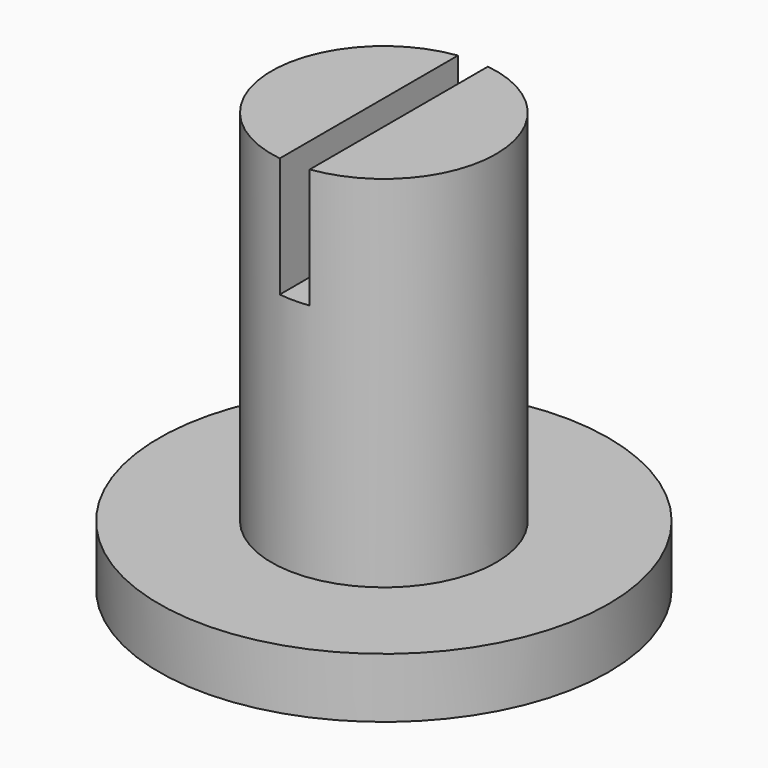
from build123d import *

# Parameters (mm, degrees)
F0_R     = 1.875
F1_DEPTH = 7
F0_R_2   = 3.75
F2_DEPTH = 1
F4_DEPTH = 2


with BuildPart() as f1:
    # F0 (on Top) → F1 (new body)
    with BuildSketch(Plane.XY):
        Circle(F0_R)
    extrude(amount=F1_DEPTH)

    # F0 (on Top) → F2 (join)
    with BuildSketch(Plane.XY):
        Circle(F0_R_2)
        Circle(F0_R, mode=Mode.SUBTRACT)
    extrude(amount=F2_DEPTH)

    # F3 (on face) → F4 (cut)
    with BuildSketch(Plane.XY.offset(7)):
        with BuildLine():
            Line((-0.25, 1.8582585934), (-0.25, -1.8582585934))
            ThreePointArc((-0.25, -1.8582585934), (0, -1.875), (0.25, -1.8582585934))
            Line((0.25, -1.8582585934), (0.25, 1.8582585934))
            ThreePointArc((0.25, 1.8582585934), (0, 1.875), (-0.25, 1.8582585934))
        make_face()
        with BuildLine():
            Line((-0.25, 2.5), (-0.25, 1.8582585934))
            ThreePointArc((-0.25, 1.8582585934), (0, 1.875), (0.25, 1.8582585934))
            Line((0.25, 1.8582585934), (0.25, 2.5))
            Line((0.25, 2.5), (-0.25, 2.5))
        make_face()
    extrude(amount=-F4_DEPTH, mode=Mode.SUBTRACT)


solid = f1.part
